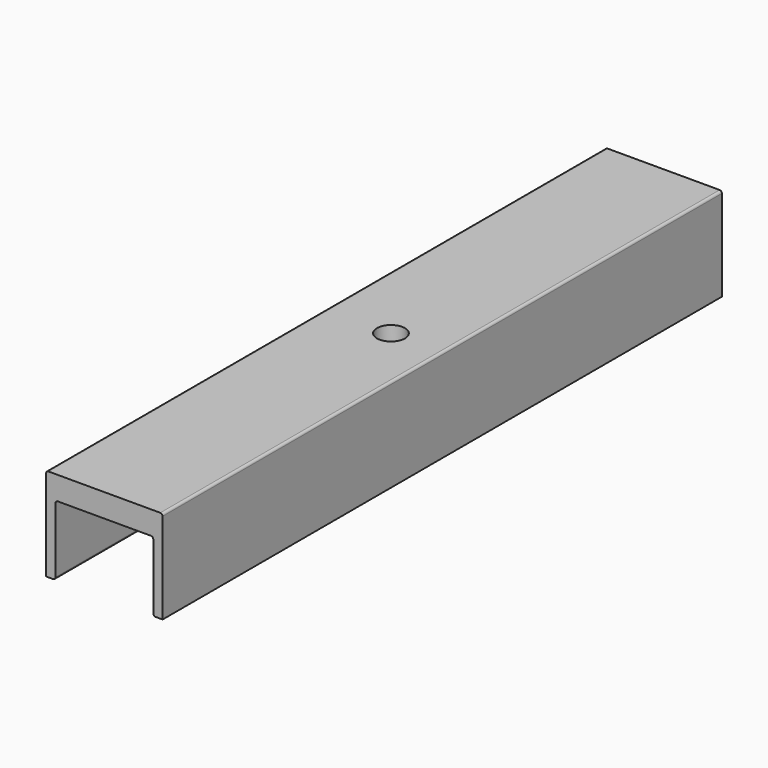
from build123d import *

# Parameters (mm, degrees)
F1_DEPTH = 75
F2_R     = 3
F3_DEPTH = 5
F4_R     = 0.5


with BuildPart() as f1:
    # F0 (on Front) → F1 (new body, symmetric)
    with BuildSketch(Plane.XZ):
        Polygon((25, 20), (0, 20), (0, 0), (2, 0), (2, 15), (23, 15), (23, 0), (25, 0), align=None)
    extrude(amount=F1_DEPTH, both=True)

    # F2 (on face) → F3 (cut, through all)
    with BuildSketch(Plane.XY.offset(20)):
        with Locations((14, 0)):
            Circle(F2_R)
    extrude(amount=-F3_DEPTH, mode=Mode.SUBTRACT)

    # F4
    f4_edges = [f1.edges().sort_by_distance(p)[0] for p in [
        (0, 0, 20),
        (25, 0, 20),
        (2, 0, 0),
        (2, 0, 15),
        (23, 0, 15),
        (23, 0, 0),
    ]]
    fillet(f4_edges, radius=F4_R)


solid = f1.part
